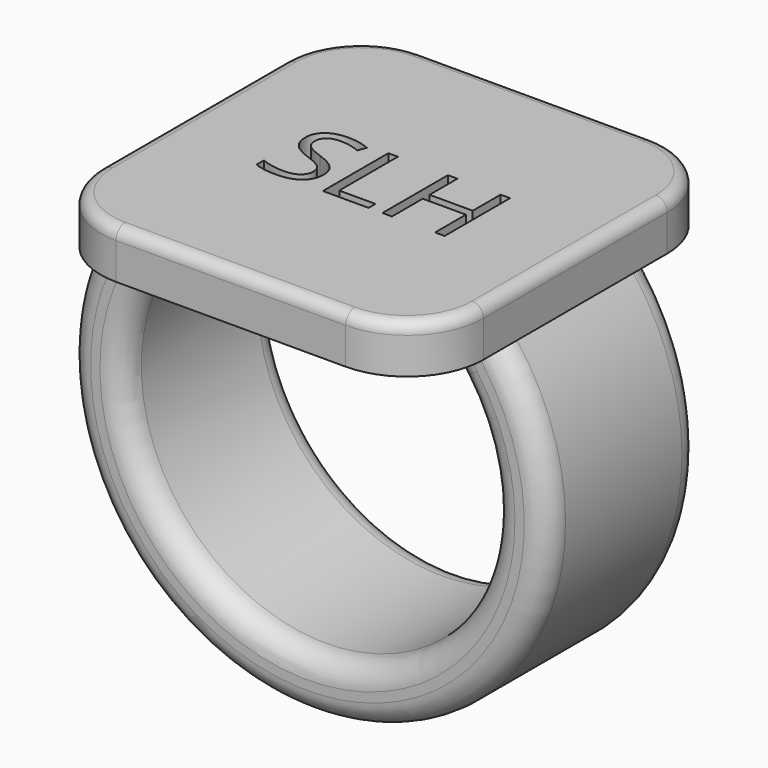
from build123d import *

# Parameters (mm, degrees)
F0_W          = 25.4
F0_H          = 25.4
F1_DEPTH      = 3.175
F3_W          = 5.08
F3_H          = 12.7
F6_DEPTH      = 6.35
F6_DEPTH_BACK = 6.35
F7_R          = 5.08
F8_R          = 1.524
F9_R          = 0.762
F10_TEXT_SIZE = 7.6134120011
F11_DEPTH     = 12.7


# Not quite as in the source:
# - Text() gives the source's letters only with a copy of the font that has no kerning and outlines rounded to 1/6400 em; it was checked with that copy


with BuildPart() as f1:
    # F0 (on Top) → F1 (new body)
    with BuildSketch(Plane.XY):
        Rectangle(F0_W, F0_H)
    extrude(amount=F1_DEPTH)

    # F4: sweep along a path in F2
    with BuildLine(Plane.XZ) as f4_path:
        ThreePointArc((-10.16, 0), (0, -23.5582897328), (10.16, 0))
    # F3 (on face) → F4 (sweep)
    with BuildSketch(Plane(origin=(0, 0, 0), x_dir=(1, 0, 0), z_dir=(0, 0, -1))):
        with Locations((-10.16, 0)):
            Rectangle(F3_W, F3_H)
    sweep(path=f4_path.line)

    # F5 (on Front) → F6 (join, two sides)
    with BuildSketch(Plane.XZ) as f6_sk:
        with BuildLine():
            ThreePointArc((7.62, 0), (8.9072265211, -1.1822790439), (10.0130578512, -2.535746045))
            Line((10.0130578512, -2.535746045), (10.16, 0))
            Line((10.16, 0), (7.62, 0))
        make_face()
    extrude(amount=F6_DEPTH)
    extrude(f6_sk.sketch, amount=-F6_DEPTH_BACK)

    # F7
    f7_edges = [f1.edges().sort_by_distance(p)[0] for p in [
        (-12.7, -12.7, 1.5875),
        (12.7, -12.7, 1.5875),
        (12.7, 12.7, 1.5875),
        (-12.7, 12.7, 1.5875),
    ]]
    fillet(f7_edges, radius=F7_R)

    # F8
    f8_edges = [f1.edges().sort_by_distance(p)[0] for p in [
        (-1.743325, 6.35, -21.711017),
        (8.907227, 6.35, -1.182279),
        (-1.743325, -6.35, -21.711017),
        (0, 6.35, -25.501344),
        (8.907227, -6.35, -1.182279),
        (0, -6.35, -25.501344),
    ]]
    fillet(f8_edges, radius=F8_R)

    # F9
    f9_edges = [f1.edges().sort_by_distance(p)[0] for p in [
        (0, -12.7, 3.175),
        (12.7, 0, 3.175),
        (11.212102, 11.212102, 3.175),
        (0, 12.7, 3.175),
        (-11.212102, 11.212102, 3.175),
        (-12.7, 0, 3.175),
        (11.212102, -11.212102, 3.175),
        (-11.212102, -11.212102, 3.175),
    ]]
    fillet(f9_edges, radius=F9_R)

    # F10 (on face) → F11 (cut)
    with BuildSketch(Plane.XY.offset(3.175)):
        with Locations((-6.7413919605, -2.8038341552)):
            Text('SLH', F10_TEXT_SIZE, font='Open Sans', text_align=(TextAlign.LEFT, TextAlign.BOTTOM))
    extrude(amount=-F11_DEPTH, mode=Mode.SUBTRACT)


solid = f1.part
